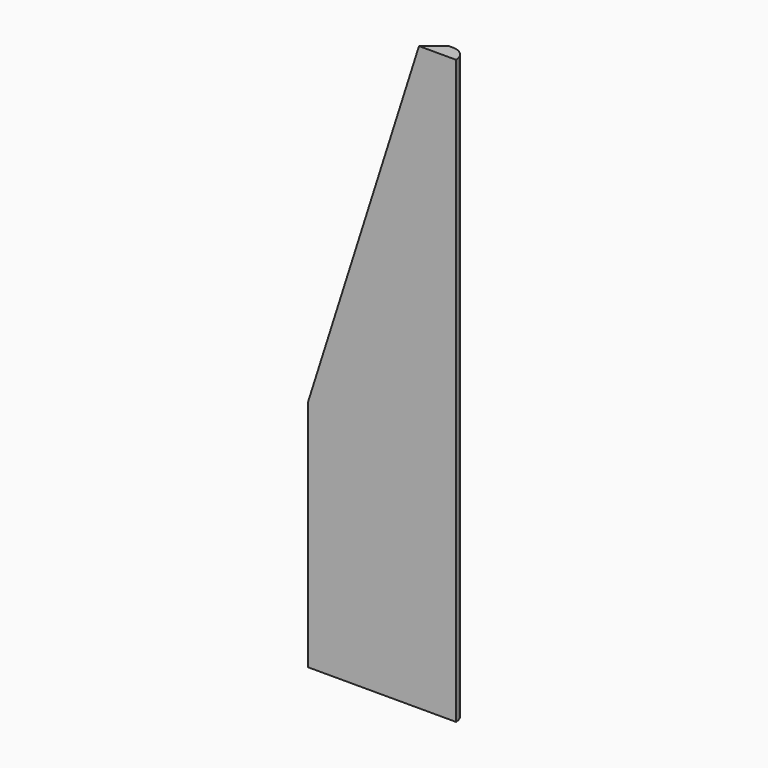
from build123d import *

# Parameters (mm, degrees)
F10_R = 2.49999


# Not quite as in the source:
# - a fillet or chamfer is up to 0.001 mm smaller than in the source, because OpenCascade refuses the exact size


with BuildPart() as f5:
    # F0 (on Top) → F5 section 0
    with BuildSketch(Plane.XY):
        Polygon((-12.7, -1.25), (12.7, -1.25), (12.7, 1.25), (0, 1.25), align=None)
    # F2 (on offset) → F5 section 1
    with BuildSketch(Plane.XY.offset(40)):
        Polygon((-12.7, -1.25), (12.7, -1.25), (12.7, 1.25), (0, 1.25), align=None)
    loft()

    # F2 (on offset) → F6 section 0
    with BuildSketch(Plane.XY.offset(40)):
        Polygon((-12.7, -1.25), (12.7, -1.25), (12.7, 1.25), (0, 1.25), align=None)
    # F4 (on offset) → F6 section 1
    with BuildSketch(Plane.XY.offset(80)):
        Polygon((0, -1.25), (12.7, -1.25), (12.7, 1.25), (6.35, 1.25), align=None)
    loft()

    # F8 (on offset) → F9 section 0
    with BuildSketch(Plane.XY.offset(100)):
        Polygon((6.35, -1.25), (12.7, -1.25), (12.7, 1.25), (9.525, 1.25), align=None)
    # F4 (on offset) → F9 section 1
    with BuildSketch(Plane.XY.offset(80)):
        Polygon((0, -1.25), (12.7, -1.25), (12.7, 1.25), (6.35, 1.25), align=None)
    loft()

    # F10 (radius 2.5 in the source; OpenCascade refuses exactly that, so slightly less here)
    f10_edges = [f5.edges().sort_by_distance(p)[0] for p in [
        (12.7, 1.25, 50),
    ]]
    fillet(f10_edges, radius=F10_R)


solid = f5.part
